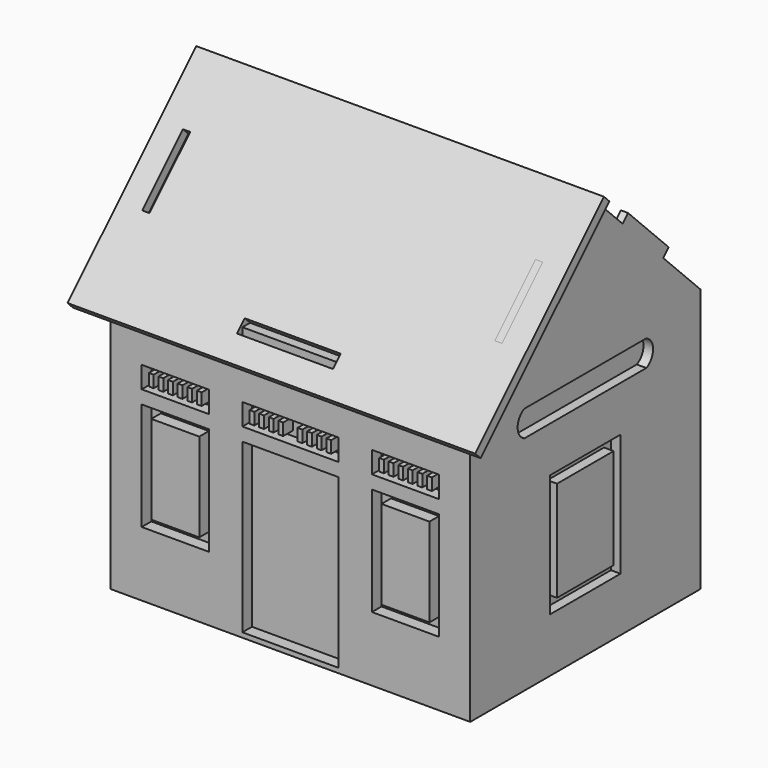
from build123d import *

# Parameters (mm, degrees)
F0_W      = 150
F0_H      = 120
F1_DEPTH  = 170
F2_SIZE   = 59.99999
F3_W      = 28
F3_H      = 9.0039297938
F3_W_2    = 2
F3_H_2    = 5.0039297938
F3_H_3    = 45
F3_W_3    = 20
F3_H_4    = 37
F3_W_4    = 40
F3_H_5    = 70
F4_DEPTH  = 5
F3_H_6    = 3.99999
F5_DEPTH  = 4
F6_W      = 36.6545170546
F6_H      = 51.0658398271
F6_W_2    = 29.4850878417
F6_H_2    = 41.9020280242
F6_W_3    = 63.571639359
F6_H_3    = 10.9027773142
F7_DEPTH  = 4
F8_DEPTH  = 3
F10_DEPTH = 4


# Not quite as in the source:
# - a fillet or chamfer is up to 0.001 mm smaller than in the source, because OpenCascade refuses the exact size
# - ends of sketch curves that miss each other by under 0.0002 mm in the source are joined
# - a feature names something its author has since deleted; it is built from what else it names


with BuildPart() as f1:
    # F0 (on Top) → F1 (new body)
    with BuildSketch(Plane.XY):
        Rectangle(F0_W, F0_H)
    extrude(amount=F1_DEPTH)

    # F2 (size 60 in the source; OpenCascade refuses exactly that, so slightly less here)
    f2_edges = [f1.edges().sort_by_distance(p)[0] for p in [
        (0, -60, 170),
        (0, 60, 170),
    ]]
    chamfer(f2_edges, length=F2_SIZE)

    # F3 (on face) → F4 (cut)
    with BuildSketch(Plane.XZ.offset(60)):
        with Locations((-48, 82.0457972586)):
            Rectangle(F3_W, F3_H)
        with Locations((-58, 82.0457972586)):
            Rectangle(F3_W_2, F3_H_2, mode=Mode.SUBTRACT)
        with Locations((-54, 82.0457972586)):
            Rectangle(F3_W_2, F3_H_2, mode=Mode.SUBTRACT)
        with Locations((-50, 82.0457972586)):
            Rectangle(F3_W_2, F3_H_2, mode=Mode.SUBTRACT)
        with Locations((-46, 82.0457972586)):
            Rectangle(F3_W_2, F3_H_2, mode=Mode.SUBTRACT)
        with Locations((-42, 82.0457972586)):
            Rectangle(F3_W_2, F3_H_2, mode=Mode.SUBTRACT)
        with Locations((-38, 82.0457972586)):
            Rectangle(F3_W_2, F3_H_2, mode=Mode.SUBTRACT)
        with Locations((-48, 49.5)):
            Rectangle(F3_W, F3_H_3)
        with Locations((-48, 49.5)):
            Rectangle(F3_W_3, F3_H_4, mode=Mode.SUBTRACT)
        with Locations((0, 37)):
            Rectangle(F3_W_4, F3_H_5)
        with Locations((0, 82.0457972586)):
            Rectangle(F3_W_4, F3_H)
        with Locations((-16, 82.0457972586)):
            Rectangle(F3_W_2, F3_H_2, mode=Mode.SUBTRACT)
        with Locations((-12, 82.0457972586)):
            Rectangle(F3_W_2, F3_H_2, mode=Mode.SUBTRACT)
        with Locations((-8, 82.0457972586)):
            Rectangle(F3_W_2, F3_H_2, mode=Mode.SUBTRACT)
        with Locations((-4, 82.0457972586)):
            Rectangle(F3_W_2, F3_H_2, mode=Mode.SUBTRACT)
        with Locations((4, 82.0457972586)):
            Rectangle(F3_W_2, F3_H_2, mode=Mode.SUBTRACT)
        with Locations((8, 82.0457972586)):
            Rectangle(F3_W_2, F3_H_2, mode=Mode.SUBTRACT)
        with Locations((12, 82.0457972586)):
            Rectangle(F3_W_2, F3_H_2, mode=Mode.SUBTRACT)
        with Locations((16, 82.0457972586)):
            Rectangle(F3_W_2, F3_H_2, mode=Mode.SUBTRACT)
        with Locations((48, 82.0457972586)):
            Rectangle(F3_W, F3_H)
        with Locations((38, 82.0457972586)):
            Rectangle(F3_W_2, F3_H_2, mode=Mode.SUBTRACT)
        with Locations((42, 82.0457972586)):
            Rectangle(F3_W_2, F3_H_2, mode=Mode.SUBTRACT)
        with Locations((46, 82.0457972586)):
            Rectangle(F3_W_2, F3_H_2, mode=Mode.SUBTRACT)
        with Locations((50, 82.0457972586)):
            Rectangle(F3_W_2, F3_H_2, mode=Mode.SUBTRACT)
        with Locations((54, 82.0457972586)):
            Rectangle(F3_W_2, F3_H_2, mode=Mode.SUBTRACT)
        with Locations((58, 82.0457972586)):
            Rectangle(F3_W_2, F3_H_2, mode=Mode.SUBTRACT)
        with Locations((48, 49.5)):
            Rectangle(F3_W, F3_H_3)
        with Locations((48, 49.5)):
            Rectangle(F3_W_3, F3_H_4, mode=Mode.SUBTRACT)
    extrude(amount=-F4_DEPTH, mode=Mode.SUBTRACT)

    # F3 (on face) → F5 (join)
    with BuildSketch(Plane.XZ.offset(60)):
        with Locations((0, 112.000005)):
            Rectangle(F3_W_4, F3_H_6)
    extrude(amount=-F5_DEPTH)

    # F6 (on face) → F7 (cut)
    with BuildSketch(Plane.YZ.offset(75)):
        with Locations((0, 48.0980910361)):
            Rectangle(F6_W, F6_H)
        with Locations((0, 48.0980910361)):
            Rectangle(F6_W_2, F6_H_2, mode=Mode.SUBTRACT)
        with Locations((0, 98.0651453137)):
            Rectangle(F6_W_3, F6_H_3)
        with BuildLine():
            Line((-31.7858196795, 92.6137566566), (-31.7858196795, 103.5165339708))
            ThreePointArc((-31.7858196795, 103.5165339708), (-35.3030027089, 98.0651453137), (-31.7858196795, 92.6137566566))
        make_face()
        with BuildLine():
            ThreePointArc((31.7858196795, 92.6137566566), (35.3030027089, 98.0651453137), (31.7858196795, 103.5165339708))
            Line((31.7858196795, 103.5165339708), (31.7858196795, 92.6137566566))
        make_face()
    extrude(amount=-F7_DEPTH, mode=Mode.SUBTRACT)

    # F6 (on face) → F8 (join)
    with BuildSketch(Plane.YZ.offset(75)):
        Polygon((-43.4350288425, 132.2218254069), (-40.6066017178, 129.3933982822), (-19.3934032822, 150.6066067178), (-22.2218254069, 153.4350288425), align=None)
        Polygon((22.2218254069, 153.4350288425), (19.3933982822, 150.6066017178), (40.6066067178, 129.3934032822), (43.4350288425, 132.2218254069), align=None)
    extrude(amount=-F8_DEPTH)


with BuildPart() as f10:
    # F9 (on face) → F10 (new body)
    with BuildSketch(Plane(origin=(0, -85, 85), x_dir=(1, 0, 0), z_dir=(0, -0.7071067812, 0.7071067812))):
        Polygon((75, 35.3553390593), (75, 62.7817459305), (72, 62.7817459305), (72, 92.7817459305), (75, 92.7817459305), (75, 120.2081528017), (-75, 120.2081528017), (-75, 92.7817459305), (-72, 92.7817459305), (-72, 62.7817459305), (-75, 62.7817459305), (-75, 35.3553390593), (-20, 35.3553390593), (-20, 41.0121933088), (20, 41.0121933088), (20, 35.3553390593), align=None)
        Polygon((75, 92.7817459305), (75, 62.7817459305), (75, 35.3553390593), (20, 35.3553390593), (-20, 35.3553390593), (-75, 35.3553390593), (-75, 62.7817459305), (-75, 92.7817459305), (-75, 120.2081528017), (-85, 120.2081528017), (-85, 25.3553390593), (0, 25.3553390593), (85, 25.3553390593), (85, 120.2081528017), (75, 120.2081528017), align=None)
    extrude(amount=F10_DEPTH)


solid = Compound([f1.part, f10.part])
